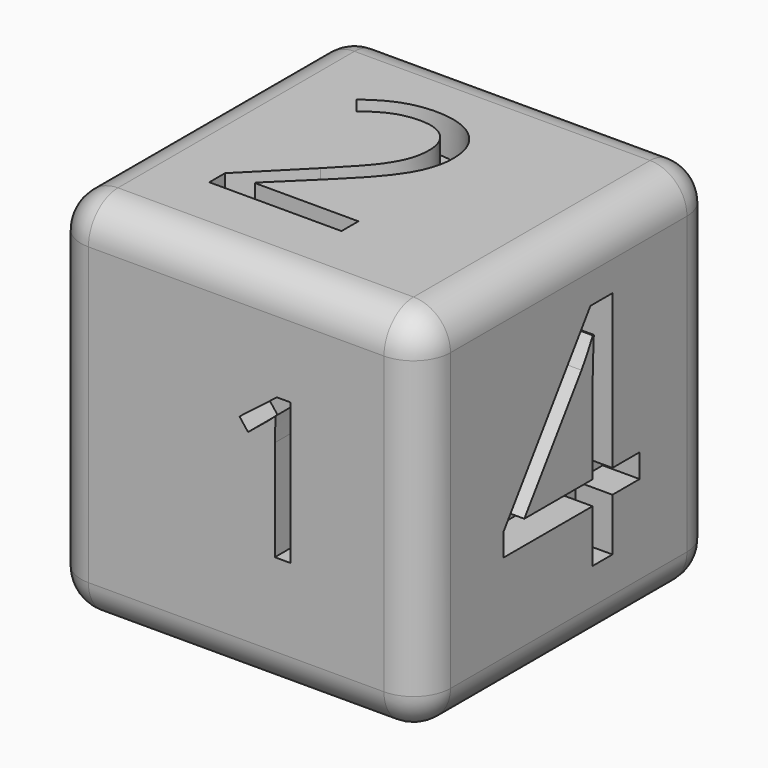
from build123d import *

# Parameters (mm, degrees)
F0_W          = 50
F0_H          = 50
F1_DEPTH      = 50
F2_R          = 5
F3_TEXT_SIZE  = 26.8099247478
F4_DEPTH      = 5
F5_TEXT_SIZE  = 39.4259142922
F6_DEPTH      = 5
F7_TEXT_SIZE  = 38.1197819176
F8_DEPTH      = 5
F9_TEXT_SIZE  = 40.4565892596
F10_DEPTH     = 5
F11_TEXT_SIZE = 35.0445295529
F12_DEPTH     = 5
F13_TEXT_SIZE = 43.3799273904
F14_DEPTH     = 5


# Not quite as in the source:
# - Text() gives the source's letters only with a copy of the font that has no kerning and outlines rounded to 1/6400 em; it was checked with that copy


with BuildPart() as f1:
    # F0 (on Front) → F1 (new body)
    with BuildSketch(Plane.XZ):
        with Locations((-9.0794473886, 10.6489803642)):
            Rectangle(F0_W, F0_H)
    extrude(amount=F1_DEPTH)

    # F2
    f2_edges = [f1.edges().sort_by_distance(p)[0] for p in [
        (-9.079447, -50, 35.64898),
        (-34.079447, -50, 10.64898),
        (-9.079447, -50, -14.35102),
        (15.920553, -50, 10.64898),
        (15.920553, -25, -14.35102),
        (15.920553, -25, 35.64898),
        (15.920553, 0, 10.64898),
        (-34.079447, -25, 35.64898),
        (-9.079447, 0, 35.64898),
        (-34.079447, 0, 10.64898),
        (-9.079447, 0, -14.35102),
        (-34.079447, -25, -14.35102),
    ]]
    fillet(f2_edges, radius=F2_R)

    # F3 (on face) → F4 (cut)
    with BuildSketch(Plane.XZ.offset(50)):
        with Locations((-11.0967954151, 1.8772883341)):
            Text('1', F3_TEXT_SIZE, font='Open Sans', text_align=(TextAlign.LEFT, TextAlign.BOTTOM))
    extrude(amount=-F4_DEPTH, mode=Mode.SUBTRACT)

    # F5 (on face) → F6 (cut)
    with BuildSketch(Plane(origin=(0, 0, 0), x_dir=(-1, 0, 0), z_dir=(0, 1, 0))):
        with Locations((-3.1273015775, -2.8862359468)):
            Text('6', F5_TEXT_SIZE, font='Open Sans', text_align=(TextAlign.LEFT, TextAlign.BOTTOM))
    extrude(amount=-F6_DEPTH, mode=Mode.SUBTRACT)

    # F7 (on face) → F8 (cut)
    with BuildSketch(Plane.XY.offset(35.6489803642)):
        with Locations((-24.206565693, -37.9718542099)):
            Text('2', F7_TEXT_SIZE, font='Open Sans', text_align=(TextAlign.LEFT, TextAlign.BOTTOM))
    extrude(amount=-F8_DEPTH, mode=Mode.SUBTRACT)

    # F9 (on face) → F10 (cut)
    with BuildSketch(Plane(origin=(0, 0, -14.3510196358), x_dir=(1, 0, 0), z_dir=(0, 0, -1))):
        with Locations((-22.5781053305, 10.9180370346)):
            Text('5', F9_TEXT_SIZE, font='Open Sans', text_align=(TextAlign.LEFT, TextAlign.BOTTOM))
    extrude(amount=-F10_DEPTH, mode=Mode.SUBTRACT)

    # F11 (on face) → F12 (cut)
    with BuildSketch(Plane(origin=(-34.0794473886, 0, 0), x_dir=(0, -1, 0), z_dir=(-1, 0, 0))):
        with Locations((9.7509361804, -1.6678082757)):
            Text('3', F11_TEXT_SIZE, font='Open Sans', text_align=(TextAlign.LEFT, TextAlign.BOTTOM))
    extrude(amount=-F12_DEPTH, mode=Mode.SUBTRACT)

    # F13 (on face) → F14 (cut)
    with BuildSketch(Plane.YZ.offset(15.9205526114)):
        with Locations((-36.9411110878, -4.5358189382)):
            Text('4', F13_TEXT_SIZE, font='Open Sans', text_align=(TextAlign.LEFT, TextAlign.BOTTOM))
    extrude(amount=-F14_DEPTH, mode=Mode.SUBTRACT)


solid = f1.part
